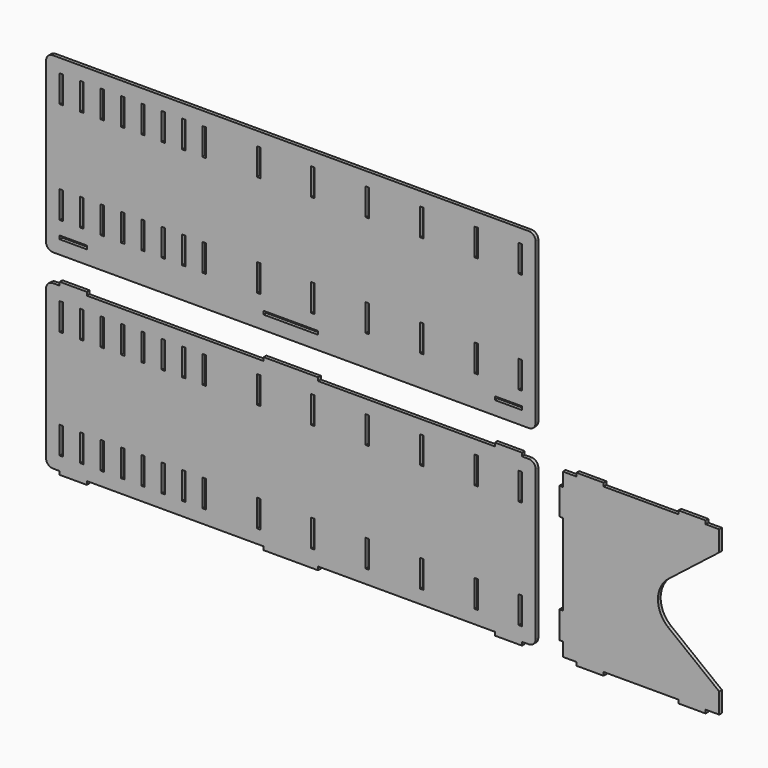
from build123d import *

# Parameters (mm, degrees)
F1_W     = 50.8
F1_H     = 6.35
F1_W_2   = 6.35
F1_H_2   = 50.8
F1_W_3   = 101.6
F2_DEPTH = 6.35


# Not quite as in the source:
# - a variable given as a bare number and used for a length is read in inches; the dataset says mm whatever the document's units were


with BuildPart() as f2:
    # F1 (on Front) → F2 (new body)
    with BuildSketch(Plane.XZ):
        with BuildLine():
            ThreePointArc((-457.2, 215.9), (-453.4802561211, 206.9197438789), (-444.5, 203.2))
            Line((-444.5, 203.2), (444.5, 203.2))
            ThreePointArc((444.5, 203.2), (453.4802561211, 206.9197438789), (457.2, 215.9))
            Line((457.2, 215.9), (457.2, 514.35))
            ThreePointArc((457.2, 514.35), (453.4802561211, 523.3302561211), (444.5, 527.05))
            Line((444.5, 527.05), (-444.5, 527.05))
            ThreePointArc((-444.5, 527.05), (-453.4802561211, 523.3302561211), (-457.2, 514.35))
            Line((-457.2, 514.35), (-457.2, 215.9))
        make_face()
        with Locations((-406.4, 231.775)):
            Rectangle(F1_W, F1_H, mode=Mode.SUBTRACT)
        with Locations((-428.625, 285.75)):
            Rectangle(F1_W_2, F1_H_2, mode=Mode.SUBTRACT)
        with Locations((-390.525, 285.75)):
            Rectangle(F1_W_2, F1_H_2, mode=Mode.SUBTRACT)
        with Locations((-352.425, 285.75)):
            Rectangle(F1_W_2, F1_H_2, mode=Mode.SUBTRACT)
        with Locations((-314.325, 285.75)):
            Rectangle(F1_W_2, F1_H_2, mode=Mode.SUBTRACT)
        with Locations((-276.225, 285.75)):
            Rectangle(F1_W_2, F1_H_2, mode=Mode.SUBTRACT)
        with Locations((-238.125, 285.75)):
            Rectangle(F1_W_2, F1_H_2, mode=Mode.SUBTRACT)
        with Locations((-200.025, 285.75)):
            Rectangle(F1_W_2, F1_H_2, mode=Mode.SUBTRACT)
        with Locations((-161.925, 285.75)):
            Rectangle(F1_W_2, F1_H_2, mode=Mode.SUBTRACT)
        with Locations((0, 231.775)):
            Rectangle(F1_W_3, F1_H, mode=Mode.SUBTRACT)
        with Locations((-60.325, 285.75)):
            Rectangle(F1_W_2, F1_H_2, mode=Mode.SUBTRACT)
        with Locations((41.275, 285.75)):
            Rectangle(F1_W_2, F1_H_2, mode=Mode.SUBTRACT)
        with Locations((142.875, 285.75)):
            Rectangle(F1_W_2, F1_H_2, mode=Mode.SUBTRACT)
        with Locations((-428.625, 476.25)):
            Rectangle(F1_W_2, F1_H_2, mode=Mode.SUBTRACT)
        with Locations((-390.525, 476.25)):
            Rectangle(F1_W_2, F1_H_2, mode=Mode.SUBTRACT)
        with Locations((-352.425, 476.25)):
            Rectangle(F1_W_2, F1_H_2, mode=Mode.SUBTRACT)
        with Locations((-314.325, 476.25)):
            Rectangle(F1_W_2, F1_H_2, mode=Mode.SUBTRACT)
        with Locations((-276.225, 476.25)):
            Rectangle(F1_W_2, F1_H_2, mode=Mode.SUBTRACT)
        with Locations((-238.125, 476.25)):
            Rectangle(F1_W_2, F1_H_2, mode=Mode.SUBTRACT)
        with Locations((-200.025, 476.25)):
            Rectangle(F1_W_2, F1_H_2, mode=Mode.SUBTRACT)
        with Locations((-161.925, 476.25)):
            Rectangle(F1_W_2, F1_H_2, mode=Mode.SUBTRACT)
        with Locations((-60.325, 476.25)):
            Rectangle(F1_W_2, F1_H_2, mode=Mode.SUBTRACT)
        with Locations((41.275, 476.25)):
            Rectangle(F1_W_2, F1_H_2, mode=Mode.SUBTRACT)
        with Locations((142.875, 476.25)):
            Rectangle(F1_W_2, F1_H_2, mode=Mode.SUBTRACT)
        with Locations((406.4, 231.775)):
            Rectangle(F1_W, F1_H, mode=Mode.SUBTRACT)
        with Locations((244.475, 285.75)):
            Rectangle(F1_W_2, F1_H_2, mode=Mode.SUBTRACT)
        with Locations((346.075, 285.75)):
            Rectangle(F1_W_2, F1_H_2, mode=Mode.SUBTRACT)
        with Locations((428.625, 285.75)):
            Rectangle(F1_W_2, F1_H_2, mode=Mode.SUBTRACT)
        with Locations((244.475, 476.25)):
            Rectangle(F1_W_2, F1_H_2, mode=Mode.SUBTRACT)
        with Locations((346.075, 476.25)):
            Rectangle(F1_W_2, F1_H_2, mode=Mode.SUBTRACT)
        with Locations((428.625, 476.25)):
            Rectangle(F1_W_2, F1_H_2, mode=Mode.SUBTRACT)
    extrude(amount=F2_DEPTH)


with BuildPart() as f2b:
    # F1 (on Front) → F2, piece 2 (new body)
    with BuildSketch(Plane.XZ):
        with BuildLine():
            Line((-431.8, 152.4), (-444.5, 152.4))
            ThreePointArc((-444.5, 152.4), (-453.4802561211, 148.6802561211), (-457.2, 139.7))
            Line((-457.2, 139.7), (-457.2, -139.7))
            ThreePointArc((-457.2, -139.7), (-453.4802561211, -148.6802561211), (-444.5, -152.4))
            Line((-444.5, -152.4), (-431.8, -152.4))
            Line((-431.8, -152.4), (-381, -152.4))
            Line((-381, -152.4), (-50.8, -152.4))
            Line((-50.8, -152.4), (50.8, -152.4))
            Line((50.8, -152.4), (381, -152.4))
            Line((381, -152.4), (431.8, -152.4))
            Line((431.8, -152.4), (444.5, -152.4))
            ThreePointArc((444.5, -152.4), (453.4802561211, -148.6802561211), (457.2, -139.7))
            Line((457.2, -139.7), (457.2, 139.7))
            ThreePointArc((457.2, 139.7), (453.4802561211, 148.6802561211), (444.5, 152.4))
            Line((444.5, 152.4), (431.8, 152.4))
            Line((431.8, 152.4), (381, 152.4))
            Line((381, 152.4), (50.8, 152.4))
            Line((50.8, 152.4), (-50.8, 152.4))
            Line((-50.8, 152.4), (-381, 152.4))
            Line((-381, 152.4), (-431.8, 152.4))
        make_face()
        with Locations((-428.625, -101.6)):
            Rectangle(F1_W_2, F1_H_2, mode=Mode.SUBTRACT)
        with Locations((-390.525, -101.6)):
            Rectangle(F1_W_2, F1_H_2, mode=Mode.SUBTRACT)
        with Locations((-352.425, -101.6)):
            Rectangle(F1_W_2, F1_H_2, mode=Mode.SUBTRACT)
        with Locations((-314.325, -101.6)):
            Rectangle(F1_W_2, F1_H_2, mode=Mode.SUBTRACT)
        with Locations((-276.225, -101.6)):
            Rectangle(F1_W_2, F1_H_2, mode=Mode.SUBTRACT)
        with Locations((-238.125, -101.6)):
            Rectangle(F1_W_2, F1_H_2, mode=Mode.SUBTRACT)
        with Locations((-200.025, -101.6)):
            Rectangle(F1_W_2, F1_H_2, mode=Mode.SUBTRACT)
        with Locations((-161.925, -101.6)):
            Rectangle(F1_W_2, F1_H_2, mode=Mode.SUBTRACT)
        with Locations((-60.325, -101.6)):
            Rectangle(F1_W_2, F1_H_2, mode=Mode.SUBTRACT)
        with Locations((41.275, -101.6)):
            Rectangle(F1_W_2, F1_H_2, mode=Mode.SUBTRACT)
        with Locations((142.875, -101.6)):
            Rectangle(F1_W_2, F1_H_2, mode=Mode.SUBTRACT)
        with Locations((-428.625, 101.6)):
            Rectangle(F1_W_2, F1_H_2, mode=Mode.SUBTRACT)
        with Locations((-390.525, 101.6)):
            Rectangle(F1_W_2, F1_H_2, mode=Mode.SUBTRACT)
        with Locations((-352.425, 101.6)):
            Rectangle(F1_W_2, F1_H_2, mode=Mode.SUBTRACT)
        with Locations((-314.325, 101.6)):
            Rectangle(F1_W_2, F1_H_2, mode=Mode.SUBTRACT)
        with Locations((-276.225, 101.6)):
            Rectangle(F1_W_2, F1_H_2, mode=Mode.SUBTRACT)
        with Locations((-238.125, 101.6)):
            Rectangle(F1_W_2, F1_H_2, mode=Mode.SUBTRACT)
        with Locations((-200.025, 101.6)):
            Rectangle(F1_W_2, F1_H_2, mode=Mode.SUBTRACT)
        with Locations((-161.925, 101.6)):
            Rectangle(F1_W_2, F1_H_2, mode=Mode.SUBTRACT)
        with Locations((-60.325, 101.6)):
            Rectangle(F1_W_2, F1_H_2, mode=Mode.SUBTRACT)
        with Locations((41.275, 101.6)):
            Rectangle(F1_W_2, F1_H_2, mode=Mode.SUBTRACT)
        with Locations((142.875, 101.6)):
            Rectangle(F1_W_2, F1_H_2, mode=Mode.SUBTRACT)
        with Locations((244.475, -101.6)):
            Rectangle(F1_W_2, F1_H_2, mode=Mode.SUBTRACT)
        with Locations((346.075, -101.6)):
            Rectangle(F1_W_2, F1_H_2, mode=Mode.SUBTRACT)
        with Locations((428.625, -101.6)):
            Rectangle(F1_W_2, F1_H_2, mode=Mode.SUBTRACT)
        with Locations((244.475, 101.6)):
            Rectangle(F1_W_2, F1_H_2, mode=Mode.SUBTRACT)
        with Locations((346.075, 101.6)):
            Rectangle(F1_W_2, F1_H_2, mode=Mode.SUBTRACT)
        with Locations((428.625, 101.6)):
            Rectangle(F1_W_2, F1_H_2, mode=Mode.SUBTRACT)
        with Locations((-406.4, 155.575)):
            Rectangle(F1_W, F1_H)
        with Locations((0, 155.575)):
            Rectangle(F1_W_3, F1_H)
        with Locations((406.4, 155.575)):
            Rectangle(F1_W, F1_H)
        with Locations((406.4, -155.575)):
            Rectangle(F1_W, F1_H)
        with Locations((0, -155.575)):
            Rectangle(F1_W_3, F1_H)
        with Locations((-406.4, -155.575)):
            Rectangle(F1_W, F1_H)
    extrude(amount=F2_DEPTH)


with BuildPart() as f2c:
    # F1 (on Front) → F2, piece 3 (new body)
    with BuildSketch(Plane.XZ):
        with Locations((558.8, 155.575)):
            Rectangle(F1_W, F1_H)
        with Locations((749.3, 155.575)):
            Rectangle(F1_W, F1_H)
        with Locations((504.825, 101.6)):
            Rectangle(F1_W_2, F1_H_2)
        with Locations((504.825, -101.6)):
            Rectangle(F1_W_2, F1_H_2)
        with BuildLine():
            Line((533.4, 152.4), (508, 152.4))
            Line((508, 152.4), (508, 127))
            Line((508, 127), (508, 76.2))
            Line((508, 76.2), (508, -76.2))
            Line((508, -76.2), (508, -127))
            Line((508, -127), (508, -152.4))
            Line((508, -152.4), (533.4, -152.4))
            Line((533.4, -152.4), (584.2, -152.4))
            Line((584.2, -152.4), (723.9, -152.4))
            Line((723.9, -152.4), (774.7, -152.4))
            Line((774.7, -152.4), (800.1, -152.4))
            Line((800.1, -152.4), (800.1, -114.3))
            Line((800.1, -114.3), (705.167824621, -40.0052540512))
            ThreePointArc((705.167824621, -40.0052540512), (685.6762843132, 0), (705.167824621, 40.0052540512))
            Line((705.167824621, 40.0052540512), (800.1, 114.3))
            Line((800.1, 114.3), (800.1, 152.4))
            Line((800.1, 152.4), (774.7, 152.4))
            Line((774.7, 152.4), (723.9, 152.4))
            Line((723.9, 152.4), (584.2, 152.4))
            Line((584.2, 152.4), (533.4, 152.4))
        make_face()
        with Locations((749.3, -155.575)):
            Rectangle(F1_W, F1_H)
        with Locations((558.8, -155.575)):
            Rectangle(F1_W, F1_H)
    extrude(amount=F2_DEPTH)


solid = Compound([f2.part, f2b.part, f2c.part])
